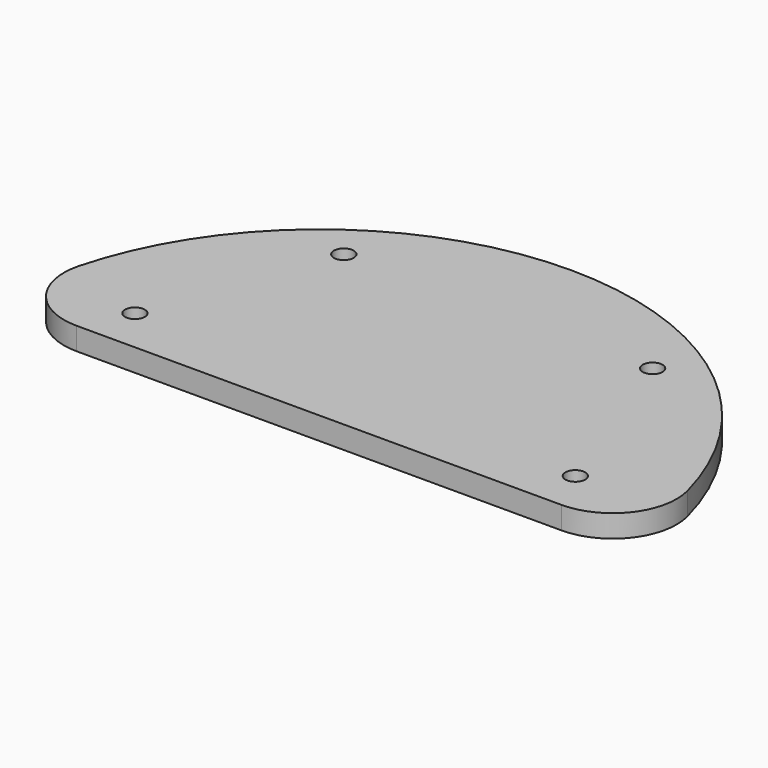
from build123d import *

# Parameters (mm, degrees)
F1_DEPTH = 5
F3_D     = 4.4
F4_R     = 14.224


with BuildPart() as f1:
    # F0 (on Top) → F1 (new body)
    with BuildSketch(Plane.XY):
        with BuildLine():
            Line((-70, 0), (70, 0))
            ThreePointArc((70, 0), (0, 70), (-70, 0))
        make_face()
    extrude(amount=F1_DEPTH)

    # F3 (through all)
    with Locations(Plane.XY.offset(5)):
        with Locations((-34.5178022981, 50), (34.1860465705, 50), (48.9897948557, 10), (-48.9897948557, 10)):
            Hole(F3_D / 2)

    # F4
    f4_edges = [f1.edges().sort_by_distance(p)[0] for p in [
        (70, 0, 2.5),
        (-70, 0, 2.5),
    ]]
    fillet(f4_edges, radius=F4_R)


solid = f1.part
